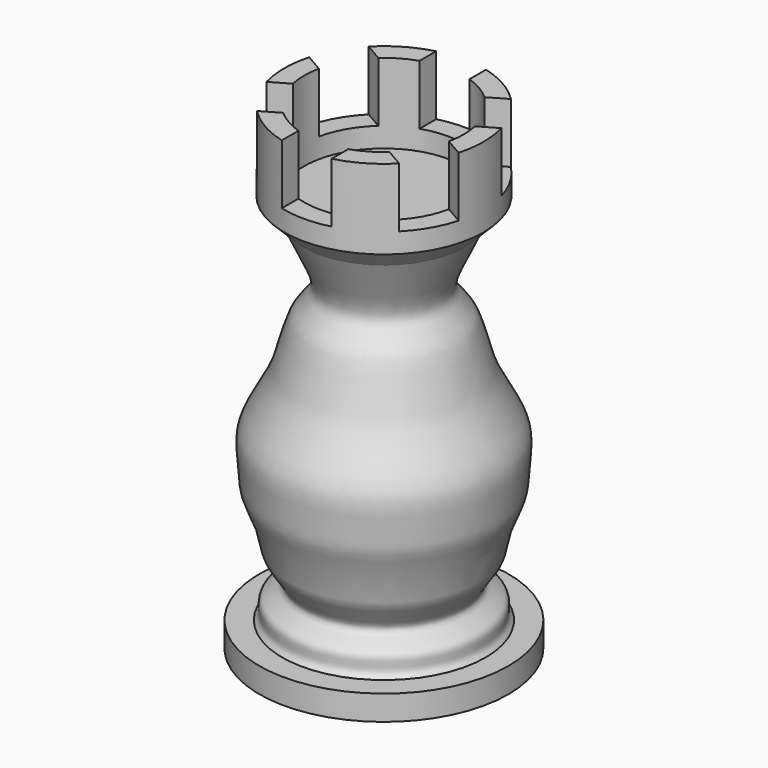
from build123d import *

# Parameters (mm, degrees)
F2_W            = 5
F2_H            = 30
F3_DEPTH        = 6
F3_COPIES_COUNT = 3
F3_COPIES_ANGLE = 120


# Not quite as in the source:
# - a pattern or mirror of a feature is missing from the dataset's text; its kind, count and spacing are read off the source's solid


with BuildPart() as f1:
    # F0 (on Front) → F1 (revolve)
    with BuildSketch(Plane.XZ):
        Polygon((0, 40), (0, 38), (8, 38), (10, 40), (10, 48), (8, 48), (8, 40), align=None)
        with BuildLine():
            Line((0, 38), (0, 2.5))
            Line((0, 2.5), (10.2003924549, 2.5))
            add(Edge.make_bspline(
                [(8, 38), (7.5248419907, 36.9634207408), (6.6072321354, 34.9616122362), (5.032155975, 31.7275294772), (7.9165360142, 29.7059480814), (8.4460306007, 24.2755860669), (12.0081386074, 19.7193012023), (11.3101289445, 16.3493559491), (11.4479534344, 13.9717045656), (9.8330891034, 11.2749850423), (9.8281818382, 8.2634857152), (6.9089904227, 5.4642589667), (10.1822771858, 4.7665875468), (9.6304944954, 3.1334674575), (10.0276999844, 2.6919555219), (10.2003924549, 2.5)],
                knots=[0, 0, 0, 0, 0.0852870265, 0.1647035607, 0.2415088177, 0.3471715334, 0.4552756797, 0.5360993675, 0.6054080845, 0.6838573716, 0.7651576552, 0.8419687707, 0.9076073475, 0.9598305767, 1, 1, 1, 1], degree=3))
            Line((8, 38), (0, 38))
        make_face()
        Polygon((0, 2.5), (0, 0), (12.5, 0), (12.5, 2.5), (10.2003924549, 2.5), align=None)
    revolve(axis=Axis((0, 0, 44), (0, 0, -1)))

    # F2 (on face) → F3 (cut)
    with BuildSketch(Plane.XY.offset(48)):
        Rectangle(F2_W, F2_H)
    f3 = extrude(amount=-F3_DEPTH, mode=Mode.SUBTRACT)

    # F3_copies: F3 ×3 about axis
    f3_copies_axis = Axis((0, 0, 0), (0, 0, 1))
    for i in range(1, F3_COPIES_COUNT):
        add(f3.rotate(f3_copies_axis, i * F3_COPIES_ANGLE / (F3_COPIES_COUNT - 1)), mode=Mode.SUBTRACT)


solid = f1.part
